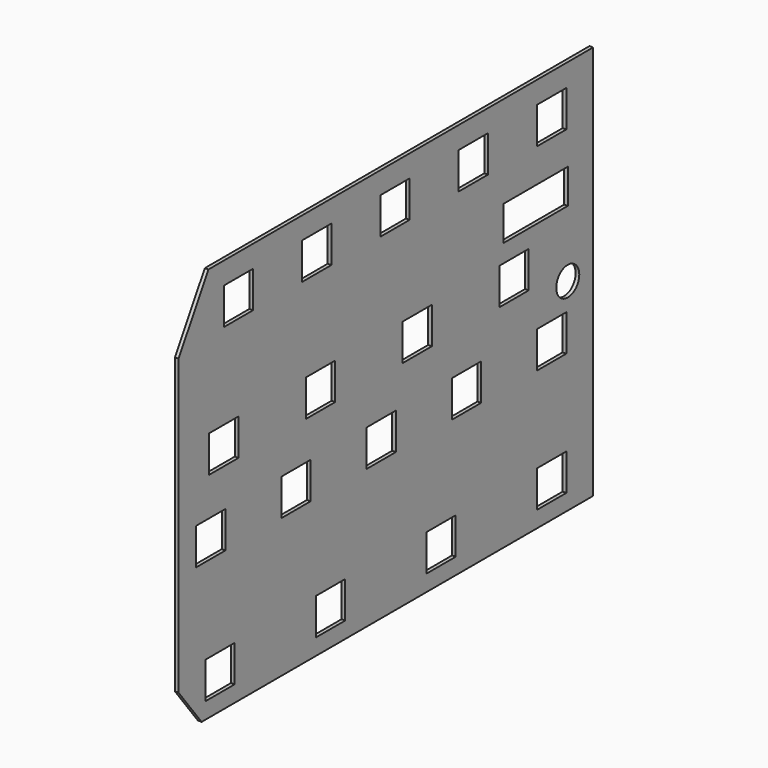
from build123d import *

# Parameters (mm, degrees)
F0_W     = 63.5
F0_H     = 63.5
F0_R     = 25
F0_W_2   = 140
F0_H_2   = 60
F1_DEPTH = 6.35


# Not quite as in the source:
# - a length typed as a fraction of an inch, garbled in the dataset ("3 / 203.2 mm" for 3/8 in), is restored


with BuildPart() as f1:
    # F0 (on Right) → F1 (new body)
    with BuildSketch(Plane.YZ):
        Polygon((-400, -342.9), (450, -342.9), (450, 342.9), (-385, 342.9), (-450, 232.9), (-450, -277.9), align=None)
        with Locations((-360, -282.9)):
            Rectangle(F0_W, F0_H, mode=Mode.SUBTRACT)
        with Locations((-120, -282.9)):
            Rectangle(F0_W, F0_H, mode=Mode.SUBTRACT)
        with Locations((-380, -70)):
            Rectangle(F0_W, F0_H, mode=Mode.SUBTRACT)
        with Locations((-195, -70)):
            Rectangle(F0_W, F0_H, mode=Mode.SUBTRACT)
        with Locations((-10, -70)):
            Rectangle(F0_W, F0_H, mode=Mode.SUBTRACT)
        with Locations((120, -282.9)):
            Rectangle(F0_W, F0_H, mode=Mode.SUBTRACT)
        with Locations((360, -282.9)):
            Rectangle(F0_W, F0_H, mode=Mode.SUBTRACT)
        with Locations((175, -70)):
            Rectangle(F0_W, F0_H, mode=Mode.SUBTRACT)
        with Locations((360, -70)):
            Rectangle(F0_W, F0_H, mode=Mode.SUBTRACT)
        with Locations((-351.75, 60)):
            Rectangle(F0_W, F0_H, mode=Mode.SUBTRACT)
        with Locations((-141.75, 60)):
            Rectangle(F0_W, F0_H, mode=Mode.SUBTRACT)
        with Locations((-320, 272.9)):
            Rectangle(F0_W, F0_H, mode=Mode.SUBTRACT)
        with Locations((-150, 272.9)):
            Rectangle(F0_W, F0_H, mode=Mode.SUBTRACT)
        with Locations((68.25, 60)):
            Rectangle(F0_W, F0_H, mode=Mode.SUBTRACT)
        with Locations((278.25, 60)):
            Rectangle(F0_W, F0_H, mode=Mode.SUBTRACT)
        with Locations((395, 7.9)):
            Circle(F0_R, mode=Mode.SUBTRACT)
        with Locations((325, 152.9)):
            Rectangle(F0_W_2, F0_H_2, mode=Mode.SUBTRACT)
        with Locations((20, 272.9)):
            Rectangle(F0_W, F0_H, mode=Mode.SUBTRACT)
        with Locations((190, 272.9)):
            Rectangle(F0_W, F0_H, mode=Mode.SUBTRACT)
        with Locations((360, 272.9)):
            Rectangle(F0_W, F0_H, mode=Mode.SUBTRACT)
    extrude(amount=F1_DEPTH)


solid = f1.part
